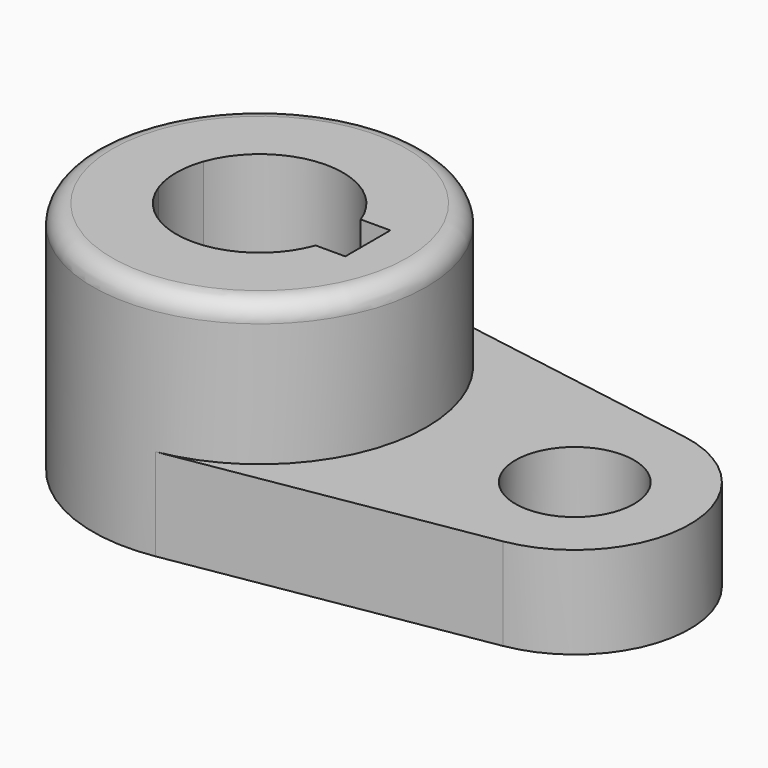
from build123d import *

# Parameters (mm, degrees)
F0_R     = 28.575
F1_DEPTH = 40.2336
F2_R     = 10.16
F3_DEPTH = 15.7734
F4_R     = 3.302


# Not quite as in the source:
# - a feature names something its author has since deleted; it is built from what else it names


with BuildPart() as f1:
    # F0 (on Top) → F1 (new body)
    with BuildSketch(Plane.XY):
        Circle(F0_R)
        with BuildLine():
            ThreePointArc((-13.4477648793, 4.826), (0, 14.2875), (13.4477648793, 4.826))
            Line((13.4477648793, 4.826), (18.5293, 4.826))
            Line((18.5293, 4.826), (18.5293, -4.826))
            Line((18.5293, -4.826), (13.4477648793, -4.826))
            ThreePointArc((13.4477648793, -4.826), (0, -14.2875), (-13.4477648793, -4.826))
            Line((-13.4477648793, -4.826), (-18.5293, -4.826))
            Line((-18.5293, -4.826), (-18.5293, 4.826))
            Line((-18.5293, 4.826), (-13.4477648793, 4.826))
        make_face(mode=Mode.SUBTRACT)
        with BuildLine():
            ThreePointArc((-13.4477648793, -4.826), (-14.2875, 0), (-13.4477648793, 4.826))
            Line((-13.4477648793, 4.826), (-18.5293, 4.826))
            Line((-18.5293, 4.826), (-18.5293, -4.826))
            Line((-18.5293, -4.826), (-13.4477648793, -4.826))
        make_face()
    extrude(amount=F1_DEPTH)

    # F2 (on Top) → F3 (join)
    with BuildSketch(Plane.XY):
        with BuildLine():
            ThreePointArc((57.2172352941, -19.4161565532), (68.9970276056, -12.7215530348), (73.66, 0))
            ThreePointArc((73.66, 0), (68.9970276056, 12.7215530348), (57.2172352941, 19.4161565532))
            ThreePointArc((57.2172352941, 19.4161565532), (34.29, 0), (57.2172352941, -19.4161565532))
        make_face()
        with Locations((53.975, 0)):
            Circle(F2_R, mode=Mode.SUBTRACT)
        with BuildLine():
            ThreePointArc((57.2172352941, -19.4161565532), (34.29, 0), (57.2172352941, 19.4161565532))
            Line((57.2172352941, 19.4161565532), (4.7064705882, 28.1847433836))
            ThreePointArc((4.7064705882, 28.1847433836), (21.8061691049, 18.4667705344), (28.575, 0))
            ThreePointArc((28.575, 0), (21.8061691049, -18.4667705344), (4.7064705882, -28.1847433836))
            Line((4.7064705882, -28.1847433836), (57.2172352941, -19.4161565532))
        make_face()
    extrude(amount=F3_DEPTH)

    # F4
    f4_edges = [f1.edges().sort_by_distance(p)[0] for p in [
        (-28.575, 0, 40.2336),
    ]]
    fillet(f4_edges, radius=F4_R)


solid = f1.part
